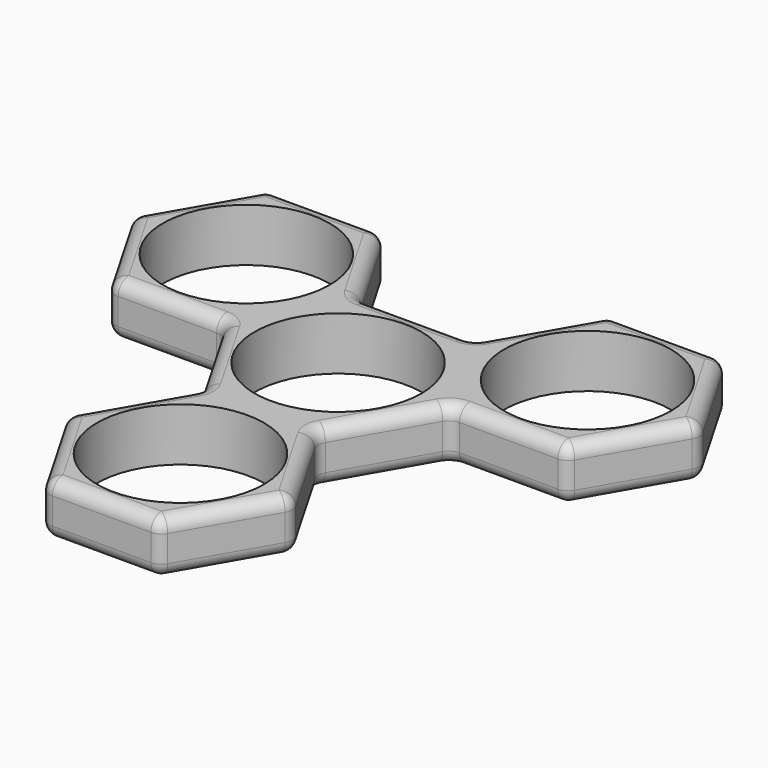
from build123d import *

# Parameters (mm, degrees)
F0_R     = 11
F1_DEPTH = 7
F2_R     = 1.75


with BuildPart() as f1:
    # F0 (on Top) → F1 (new body)
    with BuildSketch(Plane.XY):
        Polygon((15, -25.9807621135), (7.5, -12.9903810568), (-7.5, -12.9903810568), (-15, -25.9807621135), (-7.5, -38.9711431703), (7.5, -38.9711431703), align=None)
        with Locations((0, -25.9807621135)):
            Circle(F0_R, mode=Mode.SUBTRACT)
        Polygon((-7.5, -12.9903810568), (7.5, -12.9903810568), (15, 0), (7.5, 12.9903810568), (-7.5, 12.9903810568), (-15, 0), align=None)
        Circle(F0_R, mode=Mode.SUBTRACT)
        Polygon((7.5, 12.9903810568), (15, 0), (30, 0), (37.5, 12.9903810568), (30, 25.9807621135), (15, 25.9807621135), align=None)
        with Locations((22.5, 12.9903810568)):
            Circle(F0_R, mode=Mode.SUBTRACT)
        Polygon((-30, 0), (-15, 0), (-7.5, 12.9903810568), (-15, 25.9807621135), (-30, 25.9807621135), (-37.5, 12.9903810568), align=None)
        with Locations((-22.5, 12.9903810568)):
            Circle(F0_R, mode=Mode.SUBTRACT)
    extrude(amount=F1_DEPTH)

    # F2
    f2_edges = [f1.edges().sort_by_distance(p)[0] for p in [
        (7.5, -38.971143, 3.5),
        (15, -25.980762, 3.5),
        (11.25, -32.475953, 0),
        (11.25, -32.475953, 7),
        (0, -38.971143, 7),
        (11.25, -19.485572, 7),
        (11.25, -19.485572, 0),
        (11.25, -6.495191, 0),
        (7.5, -12.990381, 3.5),
        (11.25, -6.495191, 7),
        (15, 0, 3.5),
        (22.5, 0, 0),
        (22.5, 0, 7),
        (30, 0, 3.5),
        (33.75, 6.495191, 0),
        (33.75, 6.495191, 7),
        (33.75, 19.485572, 0),
        (33.75, 19.485572, 7),
        (37.5, 12.990381, 3.5),
        (30, 25.980762, 3.5),
        (22.5, 25.980762, 7),
        (22.5, 25.980762, 0),
        (11.25, 19.485572, 7),
        (11.25, 19.485572, 0),
        (0, 12.990381, 7),
        (0, 12.990381, 0),
        (-11.25, 19.485572, 7),
        (-11.25, 19.485572, 0),
        (-22.5, 25.980762, 0),
        (-15, 25.980762, 3.5),
        (-22.5, 25.980762, 7),
        (-30, 25.980762, 3.5),
        (-33.75, 19.485572, 7),
        (-33.75, 19.485572, 0),
        (-37.5, 12.990381, 3.5),
        (-33.75, 6.495191, 7),
        (-33.75, 6.495191, 0),
        (-22.5, 0, 0),
        (-30, 0, 3.5),
        (-22.5, 0, 7),
        (-15, 0, 3.5),
        (-11.25, -6.495191, 7),
        (-7.5, -12.990381, 3.5),
        (-11.25, -19.485572, 0),
        (-11.25, -19.485572, 7),
        (-15, -25.980762, 3.5),
        (-11.25, -32.475953, 7),
        (-11.25, -32.475953, 0),
        (-7.5, -38.971143, 3.5),
        (0, -38.971143, 0),
        (-7.5, 12.990381, 3.5),
        (7.5, 12.990381, 3.5),
        (15, 25.980762, 3.5),
        (-11.25, -6.495191, 0),
    ]]
    fillet(f2_edges, radius=F2_R)


solid = f1.part
